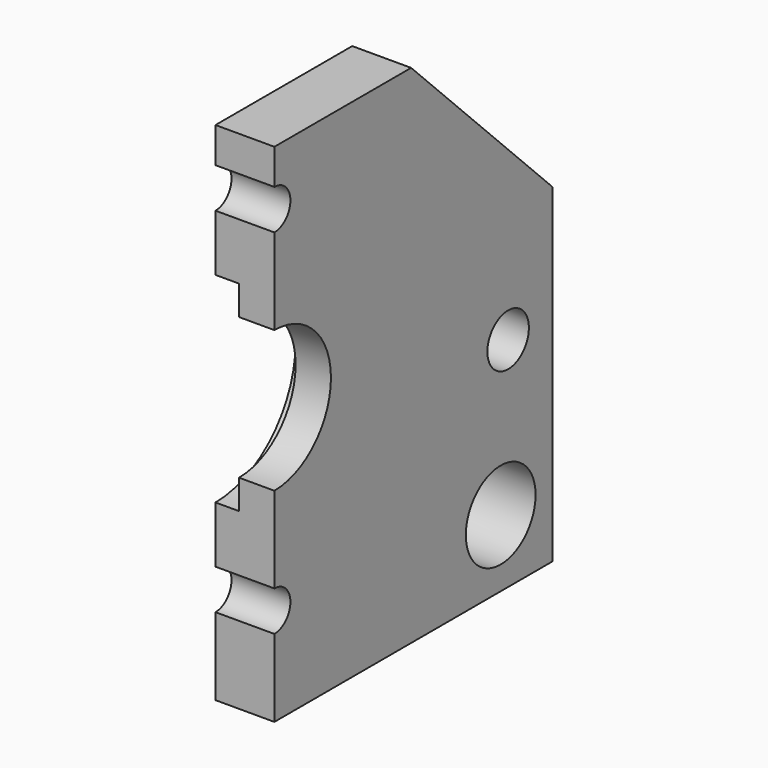
from build123d import *
from build123d import SkipClean  # not in build123d's __all__

# Parameters (mm, degrees)
F0_R     = 3.7
F0_R_2   = 2.2
F1_DEPTH = 5
F2_DEPTH = 3
F3_DEPTH = 5.001
F4_DEPTH = 2
F5_DEPTH = 2


# Not quite as in the source:
# - after a boolean that leaves OpenCascade's solid faulty, fix() repairs it
# - a feature names something its author has since deleted; it is built from what else it names


with BuildPart() as f1:
    # F0 (on Right) → F1 (new body)
    with BuildSketch(Plane.YZ):
        with BuildLine():
            Line((-33.3704365752, 11.9448962937), (-33.3704365752, 5.3711892086))
            Line((-33.3704365752, 5.3711892086), (-3.8608338702, 5.3711892086))
            Line((-3.8608338702, 5.3711892086), (-3.8608338702, 33.3448962937))
            Line((-3.8608338702, 33.3448962937), (-18.8608338702, 48.3448962937))
            Line((-18.8608338702, 48.3448962937), (-33.3704365752, 48.3448962937))
            Line((-33.3704365752, 48.3448962937), (-33.3704365752, 45.3448962937))
            ThreePointArc((-33.3704365752, 45.3448962937), (-31.6704365752, 43.6448962937), (-33.3704365752, 41.9448962937))
            Line((-33.3704365752, 41.9448962937), (-33.3704365752, 37.1448962937))
            ThreePointArc((-33.3704365752, 37.1448962937), (-24.8704365752, 28.6448962937), (-33.3704365752, 20.1448962937))
            Line((-33.3704365752, 20.1448962937), (-33.3704365752, 15.3448962937))
            ThreePointArc((-33.3704365752, 15.3448962937), (-31.6704365752, 13.6448962937), (-33.3704365752, 11.9448962937))
        make_face()
        with Locations((-9.3608338702, 11.0711892086)):
            Circle(F0_R, mode=Mode.SUBTRACT)
        with Locations((-8.5704365752, 23.8448962937)):
            Circle(F0_R_2, mode=Mode.SUBTRACT)
    extrude(amount=F1_DEPTH)

    # F0 (on Right) → F2 (join)
    with BuildSketch(Plane.YZ):
        with BuildLine():
            Line((-33.3704365752, 11.9448962937), (-33.3704365752, 5.3711892086))
            Line((-33.3704365752, 5.3711892086), (-3.8608338702, 5.3711892086))
            Line((-3.8608338702, 5.3711892086), (-3.8608338702, 33.3448962937))
            Line((-3.8608338702, 33.3448962937), (-18.8608338702, 48.3448962937))
            Line((-18.8608338702, 48.3448962937), (-33.3704365752, 48.3448962937))
            Line((-33.3704365752, 48.3448962937), (-33.3704365752, 45.3448962937))
            ThreePointArc((-33.3704365752, 45.3448962937), (-31.6704365752, 43.6448962937), (-33.3704365752, 41.9448962937))
            Line((-33.3704365752, 41.9448962937), (-33.3704365752, 37.1448962937))
            ThreePointArc((-33.3704365752, 37.1448962937), (-24.8704365752, 28.6448962937), (-33.3704365752, 20.1448962937))
            Line((-33.3704365752, 20.1448962937), (-33.3704365752, 15.3448962937))
            ThreePointArc((-33.3704365752, 15.3448962937), (-31.6704365752, 13.6448962937), (-33.3704365752, 11.9448962937))
        make_face()
        with Locations((-9.3608338702, 11.0711892086)):
            Circle(F0_R, mode=Mode.SUBTRACT)
        with Locations((-8.5704365752, 23.8448962937)):
            Circle(F0_R_2, mode=Mode.SUBTRACT)
        with BuildLine():
            Line((-33.3704365752, 15.3448962937), (-33.3704365752, 11.9448962937))
            ThreePointArc((-33.3704365752, 11.9448962937), (-31.6704365752, 13.6448962937), (-33.3704365752, 15.3448962937))
        make_face()
        with BuildLine():
            Line((-33.3704365752, 22.6448962937), (-33.3704365752, 20.1448962937))
            ThreePointArc((-33.3704365752, 20.1448962937), (-24.8704365752, 28.6448962937), (-33.3704365752, 37.1448962937))
            Line((-33.3704365752, 37.1448962937), (-33.3704365752, 34.6448962937))
            ThreePointArc((-33.3704365752, 34.6448962937), (-27.3704365752, 28.6448962937), (-33.3704365752, 22.6448962937))
        make_face()
        with BuildLine():
            Line((-33.3704365752, 34.6448962937), (-33.3704365752, 22.6448962937))
            ThreePointArc((-33.3704365752, 22.6448962937), (-27.3704365752, 28.6448962937), (-33.3704365752, 34.6448962937))
        make_face()
        with BuildLine():
            ThreePointArc((-33.3704365752, 41.9448962937), (-31.6704365752, 43.6448962937), (-33.3704365752, 45.3448962937))
            Line((-33.3704365752, 45.3448962937), (-33.3704365752, 41.9448962937))
        make_face()
    extrude(amount=F2_DEPTH)

    # F0 (on Right) → F3 (cut, through all)
    with BuildSketch(Plane.YZ):
        with BuildLine():
            Line((-33.3704365752, 34.6448962937), (-33.3704365752, 22.6448962937))
            ThreePointArc((-33.3704365752, 22.6448962937), (-27.3704365752, 28.6448962937), (-33.3704365752, 34.6448962937))
        make_face()
        with BuildLine():
            ThreePointArc((-33.3704365752, 41.9448962937), (-31.6704365752, 43.6448962937), (-33.3704365752, 45.3448962937))
            Line((-33.3704365752, 45.3448962937), (-33.3704365752, 41.9448962937))
        make_face()
        with BuildLine():
            Line((-33.3704365752, 15.3448962937), (-33.3704365752, 11.9448962937))
            ThreePointArc((-33.3704365752, 11.9448962937), (-31.6704365752, 13.6448962937), (-33.3704365752, 15.3448962937))
        make_face()
    with SkipClean():  # cleaning this boolean's faces spoils the solid; the shape is the same uncleaned
        extrude(amount=F3_DEPTH, mode=Mode.SUBTRACT)

    # F4 (add, through all): a face of the model
    f4_faces = [f1.faces().sort_by_distance(p)[0] for p in [
        (3, -25.0605023533, 28.6448962937),
    ]]
    extrude(f4_faces, amount=F4_DEPTH)

    add(f1.part.fix(), mode=Mode.REPLACE)

    # F0 (on Right) → F5 (cut)
    with BuildSketch(Plane.YZ):
        with BuildLine():
            Line((-33.3704365752, 22.6448962937), (-33.3704365752, 20.1448962937))
            ThreePointArc((-33.3704365752, 20.1448962937), (-24.8704365752, 28.6448962937), (-33.3704365752, 37.1448962937))
            Line((-33.3704365752, 37.1448962937), (-33.3704365752, 34.6448962937))
            ThreePointArc((-33.3704365752, 34.6448962937), (-27.3704365752, 28.6448962937), (-33.3704365752, 22.6448962937))
        make_face()
    extrude(amount=F5_DEPTH, mode=Mode.SUBTRACT)


solid = f1.part
